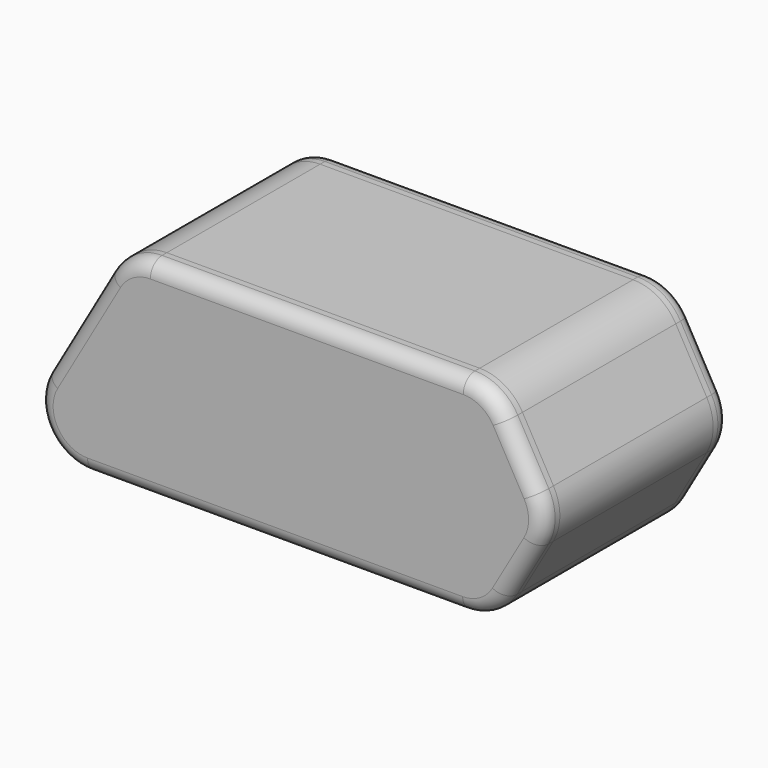
from build123d import *

# Parameters (mm, degrees)
F2_DEPTH = 65
F0_R     = 9.6692195179
F3_DEPTH = 65
F4_R     = 2
F6_DEPTH = 5
F8_DEPTH = 2
F9_R     = 5
F10_R    = 4.99999


# Not quite as in the source:
# - a fillet or chamfer is up to 0.001 mm smaller than in the source, because OpenCascade refuses the exact size


with BuildPart() as f2:
    # F1 (on Front) → F2 (new body)
    with BuildSketch(Plane.XZ):
        with BuildLine():
            Line((147.4338146996, 53.7406046613), (41.3020801363, 53.7224159943))
            ThreePointArc((41.3020801363, 53.7224159943), (32.9562626309, 51.4810350091), (26.8541756584, 45.3621304392))
            Line((26.8541756584, 45.3621304392), (5.5492387811, 8.308933718))
            ThreePointArc((5.5492387811, 8.308933718), (5.5714463746, -8.3474379072), (20, -16.6692195179))
            Line((20, -16.6692195179), (147.2401965291, -16.6692195179))
            ThreePointArc((147.2401965291, -16.6692195179), (155.574806288, -14.4359675638), (161.6761640928, -8.3346097589))
            Line((161.6761640928, -8.3346097589), (172.3777512594, 10.2010829351))
            ThreePointArc((172.3777512594, 10.2010829351), (174.6108703147, 18.4691297742), (172.4438532753, 26.7547472165))
            Line((172.4438532753, 26.7547472165), (161.9387410203, 45.2904399106))
            ThreePointArc((161.9387410203, 45.2904399106), (155.8276257555, 51.4746754645), (147.4338146996, 53.7406046613))
        make_face()
        with BuildLine():
            ThreePointArc((28.5880014327, 44.3652110923), (33.9579501109, 49.7499595653), (41.3024228927, 51.7224160237))
            Line((41.3024228927, 51.7224160237), (147.4341574561, 51.7406046906))
            ThreePointArc((147.4341574561, 51.7406046906), (154.8208654442, 49.7465453549), (160.1987591856, 44.3043044153))
            Line((160.1987591856, 44.3043044153), (170.7038714406, 25.7686117212))
            ThreePointArc((170.7038714406, 25.7686117212), (172.6108862601, 18.4771161013), (170.6457004518, 11.2010829351))
            Line((170.6457004518, 11.2010829351), (159.9441132852, -7.3346097589))
            ThreePointArc((159.9441132852, -7.3346097589), (154.574806288, -12.7039167562), (147.2401965291, -14.6692195179))
            Line((147.2401965291, -14.6692195179), (20, -14.6692195179))
            ThreePointArc((20, -14.6692195179), (7.3026076458, -7.3458987652), (7.2830645554, 7.3120143711))
            Line((7.2830645554, 7.3120143711), (28.5880014327, 44.3652110923))
        make_face(mode=Mode.SUBTRACT)
    extrude(amount=F2_DEPTH)


with BuildPart() as f3:
    # F0 (on Front) → F3 (new body)
    with BuildSketch(Plane.XZ):
        with Locations((147.2401965291, 0)):
            Circle(F0_R)
    extrude(amount=F3_DEPTH)

    # F4
    f4_edges = [f3.edges().sort_by_distance(p)[0] for p in [
        (137.570977, -65, 0),
        (137.570977, 0, 0),
    ]]
    fillet(f4_edges, radius=F4_R)


with BuildPart() as f6:
    # F5 (on face) → F6 (new body)
    with BuildSketch(Plane(origin=(0, 0, 0), x_dir=(-1, 0, 0), z_dir=(0, 1, 0))):
        with BuildLine():
            Line((-172.3777512594, 10.2010829351), (-161.6761640928, -8.3346097589))
            ThreePointArc((-161.6761640928, -8.3346097589), (-155.574806288, -14.4359675638), (-147.2401965291, -16.6692195179))
            Line((-147.2401965291, -16.6692195179), (-20, -16.6692195179))
            ThreePointArc((-20, -16.6692195179), (-5.5714463746, -8.3474379072), (-5.5492387811, 8.308933718))
            Line((-5.5492387811, 8.308933718), (-26.8541756584, 45.3621304392))
            ThreePointArc((-26.8541756584, 45.3621304392), (-32.9562626309, 51.4810350091), (-41.3020801363, 53.7224159943))
            Line((-41.3020801363, 53.7224159943), (-147.4338146996, 53.7406046613))
            ThreePointArc((-147.4338146996, 53.7406046613), (-155.8276257555, 51.4746754645), (-161.9387410203, 45.2904399106))
            Line((-161.9387410203, 45.2904399106), (-172.4438532753, 26.7547472165))
            ThreePointArc((-172.4438532753, 26.7547472165), (-174.6108703147, 18.4691297742), (-172.3777512594, 10.2010829351))
        make_face()
        with BuildLine():
            ThreePointArc((-7.2830645554, 7.3120143711), (-7.3026076458, -7.3458987652), (-20, -14.6692195179))
            Line((-20, -14.6692195179), (-147.2401965291, -14.6692195179))
            ThreePointArc((-147.2401965291, -14.6692195179), (-154.574806288, -12.7039167562), (-159.9441132852, -7.3346097589))
            Line((-159.9441132852, -7.3346097589), (-170.6457004518, 11.2010829351))
            ThreePointArc((-170.6457004518, 11.2010829351), (-172.6108862601, 18.4771161013), (-170.7038714406, 25.7686117212))
            Line((-170.7038714406, 25.7686117212), (-160.1987591856, 44.3043044153))
            ThreePointArc((-160.1987591856, 44.3043044153), (-154.8208654442, 49.7465453549), (-147.4341574561, 51.7406046906))
            Line((-147.4341574561, 51.7406046906), (-41.3024228927, 51.7224160237))
            ThreePointArc((-41.3024228927, 51.7224160237), (-33.9579501109, 49.7499595653), (-28.5880014327, 44.3652110923))
            Line((-28.5880014327, 44.3652110923), (-7.2830645554, 7.3120143711))
        make_face(mode=Mode.SUBTRACT)
    extrude(amount=F6_DEPTH)

    # F7 (on face) → F8 (join)
    with BuildSketch(Plane(origin=(0, 5, 0), x_dir=(-1, 0, 0), z_dir=(0, 1, 0))):
        with BuildLine():
            Line((-172.3777512594, 10.2010829351), (-161.6761640928, -8.3346097589))
            ThreePointArc((-161.6761640928, -8.3346097589), (-155.574806288, -14.4359675638), (-147.2401965291, -16.6692195179))
            Line((-147.2401965291, -16.6692195179), (-20, -16.6692195179))
            ThreePointArc((-20, -16.6692195179), (-5.5714463746, -8.3474379072), (-5.5492387811, 8.308933718))
            Line((-5.5492387811, 8.308933718), (-26.8541756584, 45.3621304392))
            ThreePointArc((-26.8541756584, 45.3621304392), (-32.9562626309, 51.4810350091), (-41.3020801363, 53.7224159943))
            Line((-41.3020801363, 53.7224159943), (-147.4338146996, 53.7406046613))
            ThreePointArc((-147.4338146996, 53.7406046613), (-155.8276257555, 51.4746754645), (-161.9387410203, 45.2904399106))
            Line((-161.9387410203, 45.2904399106), (-172.4438532753, 26.7547472165))
            ThreePointArc((-172.4438532753, 26.7547472165), (-174.6108703147, 18.4691297742), (-172.3777512594, 10.2010829351))
        make_face()
    extrude(amount=F8_DEPTH)

    # F9
    f9_edges = [f6.edges().sort_by_distance(p)[0] for p in [
        (167.191297, 7, 36.022594),
        (174.61087, 7, 18.46913),
        (167.026958, 7, 0.933237),
        (155.574806, 7, -14.435968),
        (83.620098, 7, -16.66922),
        (5.571446, 7, -8.347438),
        (16.201707, 7, 26.835532),
        (32.956263, 7, 51.481035),
        (94.367947, 7, 53.73151),
        (155.827626, 7, 51.474675),
    ]]
    fillet(f9_edges, radius=F9_R)

    # F10 (radius 5 in the source; OpenCascade refuses exactly that, so slightly less here)
    f10_edges = [f6.edges().sort_by_distance(p)[0] for p in [
        (33.95795, 5, 49.74996),
        (17.935533, 5, 25.838613),
        (7.302608, 5, -7.345899),
        (83.620098, 5, -14.66922),
        (154.574806, 5, -12.703917),
        (165.294907, 5, 1.933237),
        (172.610886, 5, 18.477116),
        (165.451315, 5, 35.036458),
        (154.820865, 5, 49.746545),
        (94.36829, 5, 51.73151),
    ]]
    fillet(f10_edges, radius=F10_R)


with BuildPart() as f12_1:
    # F12: instance of F6
    add(f6.part.mirror(Plane.XZ.offset(32.5)))


solid = Compound([f2.part, f3.part, f6.part, f12_1.part])
